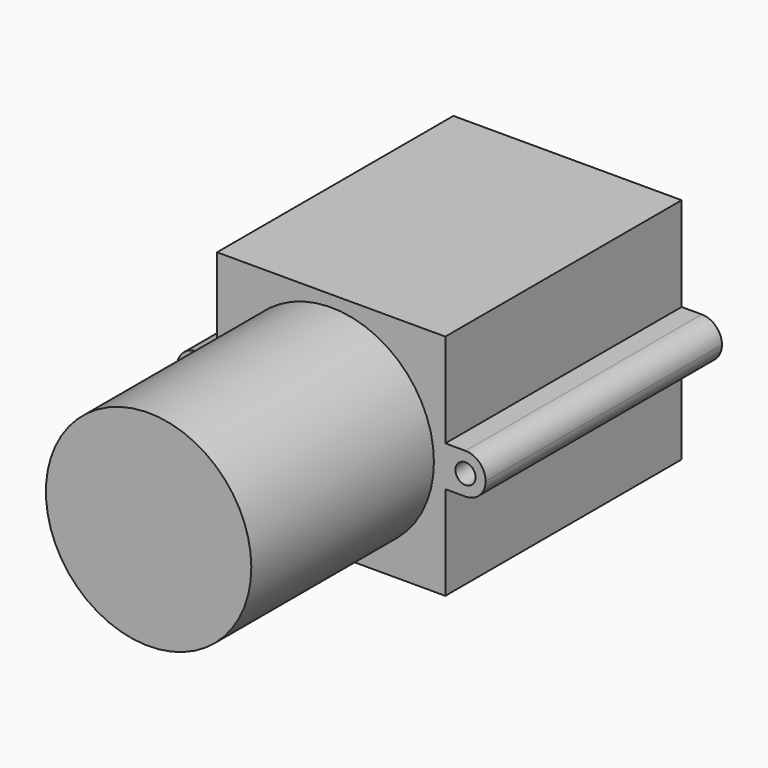
from build123d import *

# Parameters (mm, degrees)
F0_R     = 7.65
F1_DEPTH = 17
F2_W     = 17
F2_H     = 17
F3_DEPTH = 22
F4_R     = 0.75
F5_DEPTH = 22


# Not quite as in the source:
# - a pattern or mirror of a feature is missing from the dataset's text; its kind, count and spacing are read off the source's solid


with BuildPart() as f1:
    # F0 (on Front) → F1 (new body)
    with BuildSketch(Plane.XZ):
        Circle(F0_R)
    extrude(amount=F1_DEPTH)

    # F2 (on Front) → F3 (join)
    with BuildSketch(Plane.XZ):
        Rectangle(F2_W, F2_H)
    extrude(amount=-F3_DEPTH)

    # F4 (on Front) → F5 (join)
    with BuildSketch(Plane.XZ):
        with BuildLine():
            ThreePointArc((10, -1.5), (11.0606601718, -1.0606601718), (11.5, 0))
            ThreePointArc((11.5, 0), (11.0606601718, 1.0606601718), (10, 1.5))
            ThreePointArc((10, 1.5), (8.9393398282, 1.0606601718), (8.5, 0))
            ThreePointArc((8.5, 0), (8.9393398282, -1.0606601718), (10, -1.5))
        make_face()
        with Locations((10, 0)):
            Circle(F4_R, mode=Mode.SUBTRACT)
        with BuildLine():
            ThreePointArc((8.5, 0), (8.9393398282, 1.0606601718), (10, 1.5))
            Line((10, 1.5), (8.5, 1.5))
            Line((8.5, 1.5), (8.5, 0))
        make_face()
        with BuildLine():
            Line((8.5, -1.5), (10, -1.5))
            ThreePointArc((10, -1.5), (8.9393398282, -1.0606601718), (8.5, 0))
            Line((8.5, 0), (8.5, -1.5))
        make_face()
    f5 = extrude(amount=-F5_DEPTH)

    # F5_copies: F5 across plane
    add(f5.mirror(Plane(origin=(0, 0, 0), x_dir=(0, 0, -1), z_dir=(-1, 0, 0))))


solid = f1.part
